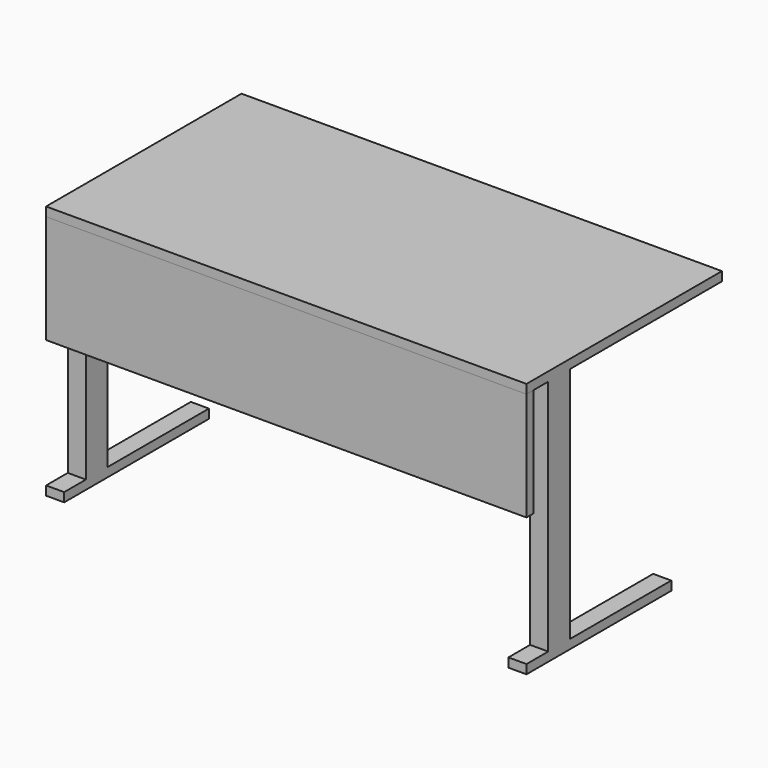
from build123d import *

# Parameters (mm, degrees)
F1_DEPTH = 25.4
F2_W     = 50.8
F2_H     = 76.2
F3_DEPTH = 685.8
F5_DEPTH = 50.8
F6_W     = 76.2
F6_H     = 21.6832172394
F7_DEPTH = 50.8
F8_W     = 1348.74
F8_H     = 304.8
F9_DEPTH = 25.4


# Not quite as in the source:
# - a feature names something its author has since deleted; it is built from what else it names


with BuildPart() as f1:
    # F0 (on Top) → F1 (new body)
    with BuildSketch(Plane.XY):
        Polygon((-75.1462131739, 533.5789480239), (-75.1462131739, -75.4217356443), (1273.5937868261, -75.4217356443), (1273.5937868261, 610.3782643557), (5.8636856265, 610.3782643557), (-75.1462131739, 610.3782643557), align=None)
    extrude(amount=F1_DEPTH)

    # F2 (on face) → F3 (join)
    with BuildSketch(Plane(origin=(0, 0, 0), x_dir=(1, 0, 0), z_dir=(0, 0, -1))):
        with Locations((-49.7462131739, -38.8782643557)):
            Rectangle(F2_W, F2_H)
        with Locations((1248.1937868261, -38.8782643557)):
            Rectangle(F2_W, F2_H)
    extrude(amount=F3_DEPTH)

    # F4 (on face) → F5 (join)
    with BuildSketch(Plane.YZ.offset(1273.5937868261)):
        Polygon((0.7782643557, -667.0380438323), (-75.4217356443, -667.0380438323), (-75.4217356443, -692.4380438323), (432.5782643557, -692.4380438323), (432.5782643557, -667.0380438323), (76.9782643557, -667.0380438323), (76.9782643557, -685.8), (0.7782643557, -685.8), align=None)
    extrude(amount=-F5_DEPTH)

    # F6 (on face) → F7 (join)
    with BuildSketch(Plane(origin=(-75.1462131739, 0, 0), x_dir=(0, -1, 0), z_dir=(-1, 0, 0))):
        with Locations((-38.8782643557, -674.9583913803)):
            Rectangle(F6_W, F6_H)
        Polygon((75.4217356443, -689.5167827606), (75.4217356443, -664.1167827606), (-0.7782643557, -664.1167827606), (-0.7782643557, -685.8), (-76.9782643557, -685.8), (-76.9782643557, -664.1167827606), (-432.5782643557, -664.1167827606), (-432.5782643557, -689.5167827606), align=None)
    extrude(amount=-F7_DEPTH)


with BuildPart() as f9:
    # F8 (on face) → F9 (new body)
    with BuildSketch(Plane.XZ.offset(75.4217356443)):
        with Locations((599.2237868261, -152.4)):
            Rectangle(F8_W, F8_H)
    extrude(amount=-F9_DEPTH)


solid = Compound([f1.part, f9.part])
